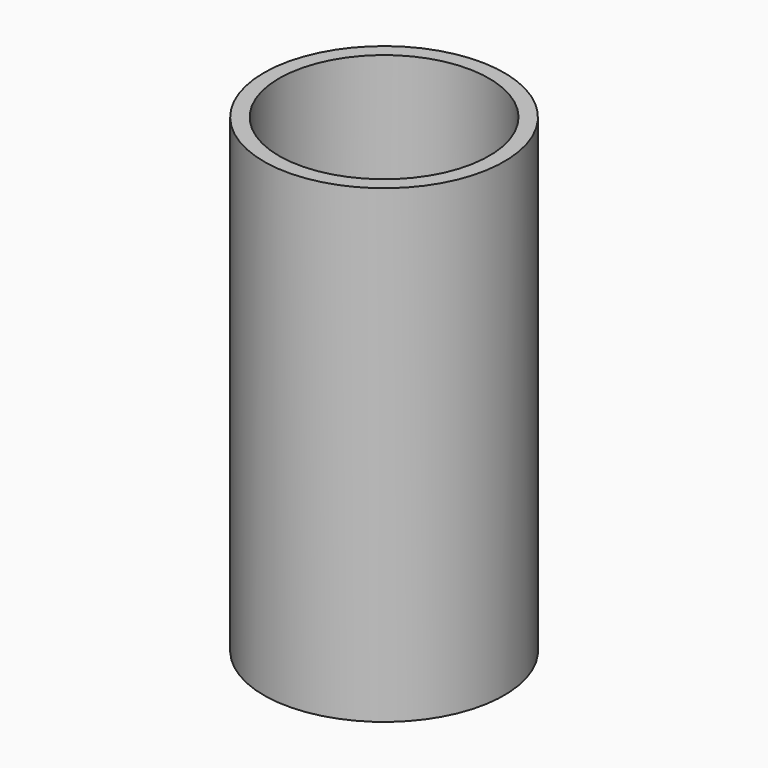
from build123d import *

# Parameters (mm, degrees)
F0_W = 20.1168013737
F0_H = 78.6383971572
F2_T = -2.54


with BuildPart() as f1:
    # F0 (on Front) → F1 (revolve)
    with BuildSketch(Plane.XZ):
        with Locations((-23.1647999026, -26.0603986681)):
            Rectangle(F0_W, F0_H)
    revolve(axis=Axis((-13.1063992158, 0, -26.0603986681), (0, 0, -1)))

    # F2
    f2_openings = [f1.faces().sort_by_distance(p)[0] for p in [
        (-13.106399, 0, 13.2588),
    ]]
    offset(amount=F2_T, openings=f2_openings)


solid = f1.part
